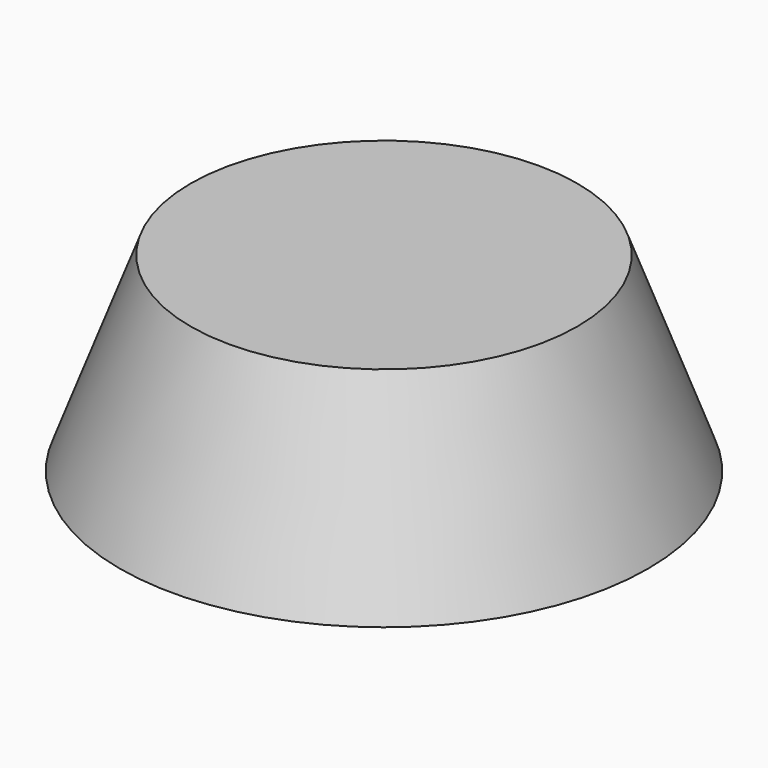
from build123d import *

# Parameters (mm, degrees)
F0_R = 35.2584515108
F2_R = 25.8270749675


with BuildPart() as f3:
    # F0 (on Top) → F3 section 0
    with BuildSketch(Plane.XY):
        Circle(F0_R)
    # F2 (on offset) → F3 section 1
    with BuildSketch(Plane.XY.offset(25.4)):
        Circle(F2_R)
    loft()


solid = f3.part
